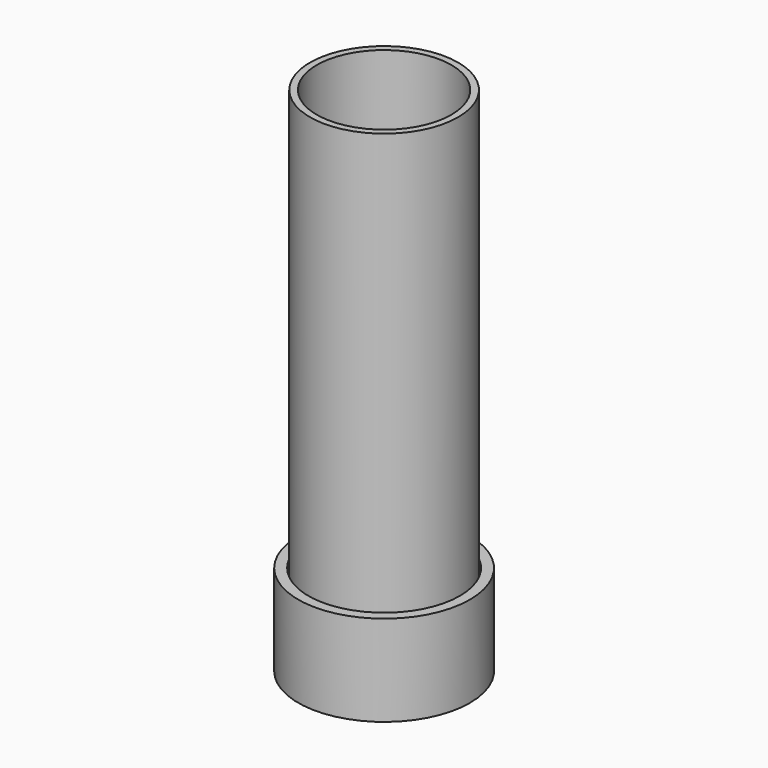
from build123d import *

# Parameters (mm, degrees)
F0_W     = 2
F0_H     = 150
F3_R     = 25.5
F3_R_2   = 22.5
F4_DEPTH = 25
F5_R     = 25.5
F6_DEPTH = 2


with BuildPart() as f1:
    # F0 (on Front) → F1 (revolve)
    with BuildSketch(Plane.XZ):
        with Locations((21, 75)):
            Rectangle(F0_W, F0_H)
    revolve(axis=Axis((0, 0, -12.3759636598), (0, 0, -1)))


with BuildPart() as f4:
    # F3 (on Top) → F4 (new body)
    with BuildSketch(Plane.XY):
        Circle(F3_R)
        Circle(F3_R_2, mode=Mode.SUBTRACT)
    extrude(amount=F4_DEPTH)

    # F5 (on face) → F6 (join)
    with BuildSketch(Plane(origin=(0, 0, 0), x_dir=(1, 0, 0), z_dir=(0, 0, -1))):
        Circle(F5_R)
    extrude(amount=F6_DEPTH)


solid = Compound([f1.part, f4.part])
